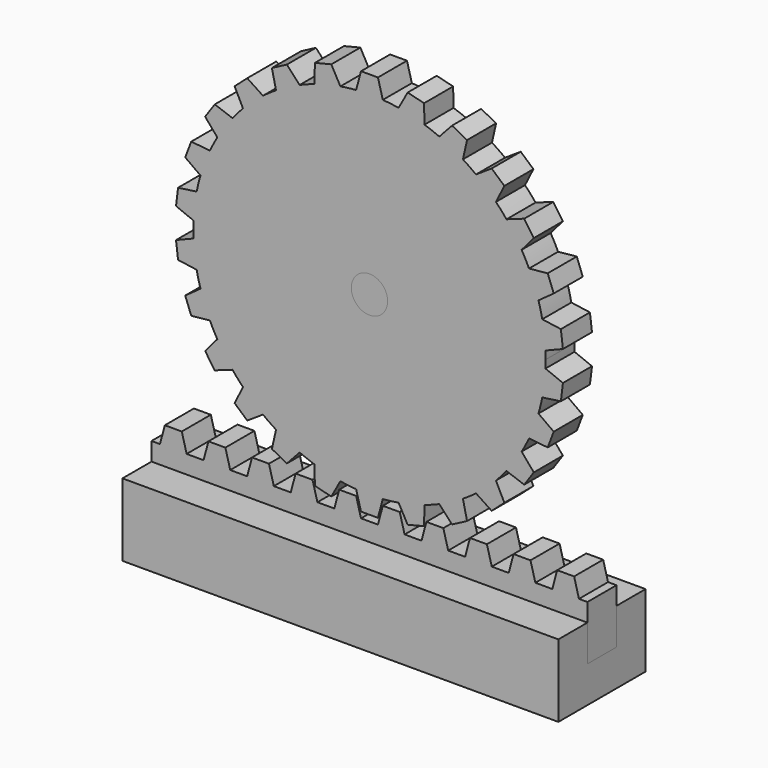
from build123d import *

# Parameters (mm, degrees)
F1_DEPTH = 12
F3_DEPTH = 2
F4_R     = 1
F5_DEPTH = 2
F6_R     = 1
F7_DEPTH = 2
F9_DEPTH = 25


with BuildPart() as f1:
    # F0 (on Right) → F1 (new body, symmetric)
    with BuildSketch(Plane.YZ):
        Polygon((0, 0), (0, 2), (-2, 2), (-2, -2), (4, -2), (4, 20), (2, 20), (2, 0), align=None)
    extrude(amount=F1_DEPTH, both=True)

    # F4 (on face) → F5 (join)
    with BuildSketch(Plane.XZ.offset(-2)):
        with Locations((0, 14)):
            Circle(F4_R)
    extrude(amount=F5_DEPTH)

    # F8 (on face) → F9 (cut)
    with BuildSketch(Plane(origin=(0, 4, 0), x_dir=(-1, 0, 0), z_dir=(0, 1, 0))):
        with BuildLine():
            Line((2, 2), (12, 2))
            Line((12, 2), (12, 20))
            Line((12, 20), (-12, 20))
            Line((-12, 20), (-12, 2))
            Line((-12, 2), (-2, 2))
            Line((-2, 2), (-2, 14))
            ThreePointArc((-2, 14), (0, 16), (2, 14))
            Line((2, 14), (2, 2))
        make_face()
    extrude(amount=-F9_DEPTH, mode=Mode.SUBTRACT)


with BuildPart() as f3:
    # F2 (on face) → F3 (new body)
    with BuildSketch(Plane.XZ.offset(-2)):
        Polygon((-12, 3), (-12, 0), (12, 0), (12, 3), (11.5339745962, 3), (11.2660254038, 4), (10.8, 4), (10.3339745962, 4), (10.0660254038, 3), (9.6, 3), (9.1339745962, 3), (8.8660254038, 4), (8.4, 4), (7.9339745962, 4), (7.6660254038, 3), (7.2, 3), (6.7339745962, 3), (6.4660254038, 4), (6, 4), (5.5339745962, 4), (5.2660254038, 3), (4.8, 3), (4.3339745962, 3), (4.0660254038, 4), (3.6, 4), (3.1339745962, 4), (2.8660254038, 3), (2.4, 3), (1.9339745962, 3), (1.6660254038, 4), (1.2, 4), (0.7339745962, 4), (0.4660254038, 3), (0, 3), (-0.4660254038, 3), (-0.7339745962, 4), (-1.2, 4), (-1.6660254038, 4), (-1.9339745962, 3), (-2.4, 3), (-2.8660254038, 3), (-3.1339745962, 4), (-3.6, 4), (-4.0660254038, 4), (-4.3339745962, 3), (-4.8, 3), (-5.2660254038, 3), (-5.5339745962, 4), (-6, 4), (-6.4660254038, 4), (-6.7339745962, 3), (-7.2, 3), (-7.6660254038, 3), (-7.9339745962, 4), (-8.4, 4), (-8.8660254038, 4), (-9.1339745962, 3), (-9.6, 3), (-10.0660254038, 3), (-10.3339745962, 4), (-10.8, 4), (-11.2660254038, 4), (-11.5339745962, 3), align=None)
    extrude(amount=F3_DEPTH)


with BuildPart() as f7:
    # F6 (on face) → F7 (new body)
    with BuildSketch(Plane.XZ.offset(-2)):
        with BuildLine():
            ThreePointArc((9.6901408298, 13.5627692852), (9.6975348942, 13.7813290707), (9.7, 14))
            ThreePointArc((9.7, 14), (9.6975348942, 14.2186709293), (9.6901408298, 14.4372307148))
            ThreePointArc((9.6901408298, 14.4372307148), (9.6292760788, 15.1692057985), (9.5131991074, 15.8944769049))
            ThreePointArc((9.5131991074, 15.8944769049), (9.418135629, 16.3213619436), (9.3039267895, 16.7435280746))
            ThreePointArc((9.3039267895, 16.7435280746), (9.069657554, 17.4396674043), (8.7833848319, 18.116084413))
            ThreePointArc((8.7833848319, 18.116084413), (8.5889234488, 18.5078147688), (8.3770023425, 18.890381555))
            ThreePointArc((8.3770023425, 18.890381555), (7.9829434992, 19.5102280433), (7.5431121563, 20.0984800563))
            ThreePointArc((7.5431121563, 20.0984800563), (7.2605542573, 20.4322897849), (6.9632369686, 20.7530238353))
            ThreePointArc((6.9632369686, 20.7530238353), (6.4322897849, 21.2605542573), (5.8644612203, 21.7264542059))
            ThreePointArc((5.8644612203, 21.7264542059), (5.5102280433, 21.9829434992), (5.1447935723, 22.2232049165))
            ThreePointArc((5.1447935723, 22.2232049165), (4.5078147688, 22.5889234488), (3.8449891145, 22.9053949216))
            ThreePointArc((3.8449891145, 22.9053949216), (3.4396674043, 23.069657554), (3.0273534742, 23.215483218))
            ThreePointArc((3.0273534742, 23.215483218), (2.3213619436, 23.418135629), (1.6020602175, 23.5667864542))
            ThreePointArc((1.6020602175, 23.5667864542), (1.1692057985, 23.6292760788), (0.7339745962, 23.6721911319))
            ThreePointArc((0.7339745962, 23.6721911319), (0, 23.7), (-0.7339745962, 23.6721911319))
            ThreePointArc((-0.7339745962, 23.6721911319), (-1.1692057985, 23.6292760788), (-1.6020602175, 23.5667864542))
            ThreePointArc((-1.6020602175, 23.5667864542), (-2.3213619436, 23.418135629), (-3.0273534742, 23.215483218))
            ThreePointArc((-3.0273534742, 23.215483218), (-3.4396674043, 23.069657554), (-3.8449891145, 22.9053949216))
            ThreePointArc((-3.8449891145, 22.9053949216), (-4.5078147688, 22.5889234488), (-5.1447935723, 22.2232049165))
            ThreePointArc((-5.1447935723, 22.2232049165), (-5.5102280433, 21.9829434992), (-5.8644612203, 21.7264542059))
            ThreePointArc((-5.8644612203, 21.7264542059), (-6.4322897849, 21.2605542573), (-6.9632369686, 20.7530238353))
            ThreePointArc((-6.9632369686, 20.7530238353), (-7.2605542573, 20.4322897849), (-7.5431121563, 20.0984800563))
            ThreePointArc((-7.5431121563, 20.0984800563), (-7.9829434992, 19.5102280433), (-8.3770023425, 18.890381555))
            ThreePointArc((-8.3770023425, 18.890381555), (-8.5889234488, 18.5078147688), (-8.7833848319, 18.116084413))
            ThreePointArc((-8.7833848319, 18.116084413), (-9.069657554, 17.4396674043), (-9.3039267895, 16.7435280746))
            ThreePointArc((-9.3039267895, 16.7435280746), (-9.418135629, 16.3213619436), (-9.5131991074, 15.8944769049))
            ThreePointArc((-9.5131991074, 15.8944769049), (-9.6292760788, 15.1692057985), (-9.6901408298, 14.4372307148))
            ThreePointArc((-9.6901408298, 14.4372307148), (-9.7, 14), (-9.6901408298, 13.5627692852))
            ThreePointArc((-9.6901408298, 13.5627692852), (-9.6292760788, 12.8307942015), (-9.5131991074, 12.1055230951))
            ThreePointArc((-9.5131991074, 12.1055230951), (-9.418135629, 11.6786380564), (-9.3039267895, 11.2564719254))
            ThreePointArc((-9.3039267895, 11.2564719254), (-9.069657554, 10.5603325957), (-8.7833848319, 9.883915587))
            ThreePointArc((-8.7833848319, 9.883915587), (-8.5889234488, 9.4921852312), (-8.3770023425, 9.109618445))
            ThreePointArc((-8.3770023425, 9.109618445), (-7.9829434992, 8.4897719567), (-7.5431121563, 7.9015199437))
            ThreePointArc((-7.5431121563, 7.9015199437), (-7.2605542573, 7.5677102151), (-6.9632369686, 7.2469761647))
            ThreePointArc((-6.9632369686, 7.2469761647), (-6.4322897849, 6.7394457427), (-5.8644612203, 6.2735457941))
            ThreePointArc((-5.8644612203, 6.2735457941), (-5.5102280433, 6.0170565008), (-5.1447935723, 5.7767950835))
            ThreePointArc((-5.1447935723, 5.7767950835), (-4.5078147688, 5.4110765512), (-3.8449891145, 5.0946050784))
            ThreePointArc((-3.8449891145, 5.0946050784), (-3.4396674043, 4.930342446), (-3.0273534742, 4.784516782))
            ThreePointArc((-3.0273534742, 4.784516782), (-2.3213619436, 4.581864371), (-1.6020602175, 4.4332135458))
            ThreePointArc((-1.6020602175, 4.4332135458), (-1.1692057985, 4.3707239212), (-0.7339745962, 4.3278088681))
            ThreePointArc((-0.7339745962, 4.3278088681), (0, 4.3), (0.7339745962, 4.3278088681))
            ThreePointArc((0.7339745962, 4.3278088681), (1.1692057985, 4.3707239212), (1.6020602175, 4.4332135458))
            ThreePointArc((1.6020602175, 4.4332135458), (2.3213619436, 4.581864371), (3.0273534742, 4.784516782))
            ThreePointArc((3.0273534742, 4.784516782), (3.4396674043, 4.930342446), (3.8449891145, 5.0946050784))
            ThreePointArc((3.8449891145, 5.0946050784), (4.5078147688, 5.4110765512), (5.1447935723, 5.7767950835))
            ThreePointArc((5.1447935723, 5.7767950835), (5.5102280433, 6.0170565008), (5.8644612203, 6.2735457941))
            ThreePointArc((5.8644612203, 6.2735457941), (6.4322897849, 6.7394457427), (6.9632369686, 7.2469761647))
            ThreePointArc((6.9632369686, 7.2469761647), (7.2605542573, 7.5677102151), (7.5431121563, 7.9015199437))
            ThreePointArc((7.5431121563, 7.9015199437), (7.9829434992, 8.4897719567), (8.3770023425, 9.109618445))
            ThreePointArc((8.3770023425, 9.109618445), (8.5889234488, 9.4921852312), (8.7833848319, 9.883915587))
            ThreePointArc((8.7833848319, 9.883915587), (9.069657554, 10.5603325957), (9.3039267895, 11.2564719254))
            ThreePointArc((9.3039267895, 11.2564719254), (9.418135629, 11.6786380564), (9.5131991074, 12.1055230951))
            ThreePointArc((9.5131991074, 12.1055230951), (9.6292760788, 12.8307942015), (9.6901408298, 13.5627692852))
        make_face()
        with Locations((0, 14)):
            Circle(F6_R, mode=Mode.SUBTRACT)
        with BuildLine():
            ThreePointArc((9.5131991074, 15.8944769049), (9.6292760788, 15.1692057985), (9.6901408298, 14.4372307148))
            Line((9.6901408298, 14.4372307148), (10.6505519978, 14.8237629362))
            Line((10.6505519978, 14.8237629362), (10.5382056876, 15.749018044))
            Line((10.5382056876, 15.749018044), (9.5131991074, 15.8944769049))
        make_face()
        with BuildLine():
            Line((10.6505519978, 13.1762370638), (9.6901408298, 13.5627692852))
            ThreePointArc((9.6901408298, 13.5627692852), (9.6292760788, 12.8307942015), (9.5131991074, 12.1055230951))
            Line((9.5131991074, 12.1055230951), (10.5382056876, 12.250981956))
            Line((10.5382056876, 12.250981956), (10.6505519978, 13.1762370638))
        make_face()
        with BuildLine():
            ThreePointArc((8.7833848319, 18.116084413), (9.069657554, 17.4396674043), (9.3039267895, 16.7435280746))
            Line((9.3039267895, 16.7435280746), (10.143926939, 17.3486698088))
            Line((10.143926939, 17.3486698088), (9.8134171677, 18.2201524529))
            Line((9.8134171677, 18.2201524529), (8.7833848319, 18.116084413))
        make_face()
        with BuildLine():
            Line((10.143926939, 10.6513301912), (9.3039267895, 11.2564719254))
            ThreePointArc((9.3039267895, 11.2564719254), (9.069657554, 10.5603325957), (8.7833848319, 9.883915587))
            Line((8.7833848319, 9.883915587), (9.8134171677, 9.7798475471))
            Line((9.8134171677, 9.7798475471), (10.143926939, 10.6513301912))
        make_face()
        with BuildLine():
            ThreePointArc((7.5431121563, 20.0984800563), (7.9829434992, 19.5102280433), (8.3770023425, 18.890381555))
            Line((8.3770023425, 18.890381555), (9.0477737183, 19.678964164))
            Line((9.0477737183, 19.678964164), (8.5183085123, 20.4460269408))
            Line((8.5183085123, 20.4460269408), (7.5431121563, 20.0984800563))
        make_face()
        with BuildLine():
            Line((9.0477737183, 8.321035836), (8.3770023425, 9.109618445))
            ThreePointArc((8.3770023425, 9.109618445), (7.9829434992, 8.4897719567), (7.5431121563, 7.9015199437))
            Line((7.5431121563, 7.9015199437), (8.5183085123, 7.5539730592))
            Line((8.5183085123, 7.5539730592), (9.0477737183, 8.321035836))
        make_face()
        with BuildLine():
            ThreePointArc((5.8644612203, 21.7264542059), (6.4322897849, 21.2605542573), (6.9632369686, 20.7530238353))
            Line((6.9632369686, 20.7530238353), (7.4257967763, 21.6792177642))
            Line((7.4257967763, 21.6792177642), (6.728146729, 22.2972817733))
            Line((6.728146729, 22.2972817733), (5.8644612203, 21.7264542059))
        make_face()
        with BuildLine():
            Line((7.4257967763, 6.3207822358), (6.9632369686, 7.2469761647))
            ThreePointArc((6.9632369686, 7.2469761647), (6.4322897849, 6.7394457427), (5.8644612203, 6.2735457941))
            Line((5.8644612203, 6.2735457941), (6.728146729, 5.7027182267))
            Line((6.728146729, 5.7027182267), (7.4257967763, 6.3207822358))
        make_face()
        with BuildLine():
            ThreePointArc((3.8449891145, 22.9053949216), (4.5078147688, 22.5889234488), (5.1447935723, 22.2232049165))
            Line((5.1447935723, 22.2232049165), (5.3722595174, 23.2331831408))
            Line((5.3722595174, 23.2331831408), (4.5469695136, 23.6663287486))
            Line((4.5469695136, 23.6663287486), (3.8449891145, 22.9053949216))
        make_face()
        with BuildLine():
            Line((5.3722595174, 4.7668168592), (5.1447935723, 5.7767950835))
            ThreePointArc((5.1447935723, 5.7767950835), (4.5078147688, 5.4110765512), (3.8449891145, 5.0946050784))
            Line((3.8449891145, 5.0946050784), (4.5469695136, 4.3336712514))
            Line((4.5469695136, 4.3336712514), (5.3722595174, 4.7668168592))
        make_face()
        with BuildLine():
            ThreePointArc((1.6020602175, 23.5667864542), (2.3213619436, 23.418135629), (3.0273534742, 23.215483218))
            Line((3.0273534742, 23.215483218), (3.0065060627, 24.2505494744))
            Line((3.0065060627, 24.2505494744), (2.1015389576, 24.4736038326))
            Line((2.1015389576, 24.4736038326), (1.6020602175, 23.5667864542))
        make_face()
        with BuildLine():
            Line((3.0065060627, 3.7494505256), (3.0273534742, 4.784516782))
            ThreePointArc((3.0273534742, 4.784516782), (2.3213619436, 4.581864371), (1.6020602175, 4.4332135458))
            Line((1.6020602175, 4.4332135458), (2.1015389576, 3.5263961674))
            Line((2.1015389576, 3.5263961674), (3.0065060627, 3.7494505256))
        make_face()
        with BuildLine():
            ThreePointArc((-0.7339745962, 23.6721911319), (0, 23.7), (0.7339745962, 23.6721911319))
            Line((0.7339745962, 23.6721911319), (0.4660254038, 24.6721911319))
            Line((0.4660254038, 24.6721911319), (-0.4660254038, 24.6721911319))
            Line((-0.4660254038, 24.6721911319), (-0.7339745962, 23.6721911319))
        make_face()
        with BuildLine():
            Line((0.4660254038, 3.3278088681), (0.7339745962, 4.3278088681))
            ThreePointArc((0.7339745962, 4.3278088681), (0, 4.3), (-0.7339745962, 4.3278088681))
            Line((-0.7339745962, 4.3278088681), (-0.4660254038, 3.3278088681))
            Line((-0.4660254038, 3.3278088681), (0.4660254038, 3.3278088681))
        make_face()
        with BuildLine():
            ThreePointArc((-3.0273534742, 23.215483218), (-2.3213619436, 23.418135629), (-1.6020602175, 23.5667864542))
            Line((-1.6020602175, 23.5667864542), (-2.1015389576, 24.4736038326))
            Line((-2.1015389576, 24.4736038326), (-3.0065060627, 24.2505494744))
            Line((-3.0065060627, 24.2505494744), (-3.0273534742, 23.215483218))
        make_face()
        with BuildLine():
            Line((-2.1015389576, 3.5263961674), (-1.6020602175, 4.4332135458))
            ThreePointArc((-1.6020602175, 4.4332135458), (-2.3213619436, 4.581864371), (-3.0273534742, 4.784516782))
            Line((-3.0273534742, 4.784516782), (-3.0065060627, 3.7494505256))
            Line((-3.0065060627, 3.7494505256), (-2.1015389576, 3.5263961674))
        make_face()
        with BuildLine():
            ThreePointArc((-5.1447935723, 22.2232049165), (-4.5078147688, 22.5889234488), (-3.8449891145, 22.9053949216))
            Line((-3.8449891145, 22.9053949216), (-4.5469695136, 23.6663287486))
            Line((-4.5469695136, 23.6663287486), (-5.3722595174, 23.2331831408))
            Line((-5.3722595174, 23.2331831408), (-5.1447935723, 22.2232049165))
        make_face()
        with BuildLine():
            Line((-4.5469695136, 4.3336712514), (-3.8449891145, 5.0946050784))
            ThreePointArc((-3.8449891145, 5.0946050784), (-4.5078147688, 5.4110765512), (-5.1447935723, 5.7767950835))
            Line((-5.1447935723, 5.7767950835), (-5.3722595174, 4.7668168592))
            Line((-5.3722595174, 4.7668168592), (-4.5469695136, 4.3336712514))
        make_face()
        with BuildLine():
            ThreePointArc((-6.9632369686, 20.7530238353), (-6.4322897849, 21.2605542573), (-5.8644612203, 21.7264542059))
            Line((-5.8644612203, 21.7264542059), (-6.728146729, 22.2972817733))
            Line((-6.728146729, 22.2972817733), (-7.4257967763, 21.6792177642))
            Line((-7.4257967763, 21.6792177642), (-6.9632369686, 20.7530238353))
        make_face()
        with BuildLine():
            Line((-6.728146729, 5.7027182267), (-5.8644612203, 6.2735457941))
            ThreePointArc((-5.8644612203, 6.2735457941), (-6.4322897849, 6.7394457427), (-6.9632369686, 7.2469761647))
            Line((-6.9632369686, 7.2469761647), (-7.4257967763, 6.3207822358))
            Line((-7.4257967763, 6.3207822358), (-6.728146729, 5.7027182267))
        make_face()
        with BuildLine():
            ThreePointArc((-8.3770023425, 18.890381555), (-7.9829434992, 19.5102280433), (-7.5431121563, 20.0984800563))
            Line((-7.5431121563, 20.0984800563), (-8.5183085123, 20.4460269408))
            Line((-8.5183085123, 20.4460269408), (-9.0477737183, 19.678964164))
            Line((-9.0477737183, 19.678964164), (-8.3770023425, 18.890381555))
        make_face()
        with BuildLine():
            Line((-8.5183085123, 7.5539730592), (-7.5431121563, 7.9015199437))
            ThreePointArc((-7.5431121563, 7.9015199437), (-7.9829434992, 8.4897719567), (-8.3770023425, 9.109618445))
            Line((-8.3770023425, 9.109618445), (-9.0477737183, 8.321035836))
            Line((-9.0477737183, 8.321035836), (-8.5183085123, 7.5539730592))
        make_face()
        with BuildLine():
            ThreePointArc((-9.3039267895, 16.7435280746), (-9.069657554, 17.4396674043), (-8.7833848319, 18.116084413))
            Line((-8.7833848319, 18.116084413), (-9.8134171677, 18.2201524529))
            Line((-9.8134171677, 18.2201524529), (-10.143926939, 17.3486698088))
            Line((-10.143926939, 17.3486698088), (-9.3039267895, 16.7435280746))
        make_face()
        with BuildLine():
            Line((-9.8134171677, 9.7798475471), (-8.7833848319, 9.883915587))
            ThreePointArc((-8.7833848319, 9.883915587), (-9.069657554, 10.5603325957), (-9.3039267895, 11.2564719254))
            Line((-9.3039267895, 11.2564719254), (-10.143926939, 10.6513301912))
            Line((-10.143926939, 10.6513301912), (-9.8134171677, 9.7798475471))
        make_face()
        with BuildLine():
            ThreePointArc((-9.6901408298, 14.4372307148), (-9.6292760788, 15.1692057985), (-9.5131991074, 15.8944769049))
            Line((-9.5131991074, 15.8944769049), (-10.5382056876, 15.749018044))
            Line((-10.5382056876, 15.749018044), (-10.6505519978, 14.8237629362))
            Line((-10.6505519978, 14.8237629362), (-9.6901408298, 14.4372307148))
        make_face()
        with BuildLine():
            Line((-10.5382056876, 12.250981956), (-9.5131991074, 12.1055230951))
            ThreePointArc((-9.5131991074, 12.1055230951), (-9.6292760788, 12.8307942015), (-9.6901408298, 13.5627692852))
            Line((-9.6901408298, 13.5627692852), (-10.6505519978, 13.1762370638))
            Line((-10.6505519978, 13.1762370638), (-10.5382056876, 12.250981956))
        make_face()
    extrude(amount=F7_DEPTH)


solid = Compound([f1.part, f3.part, f7.part])
